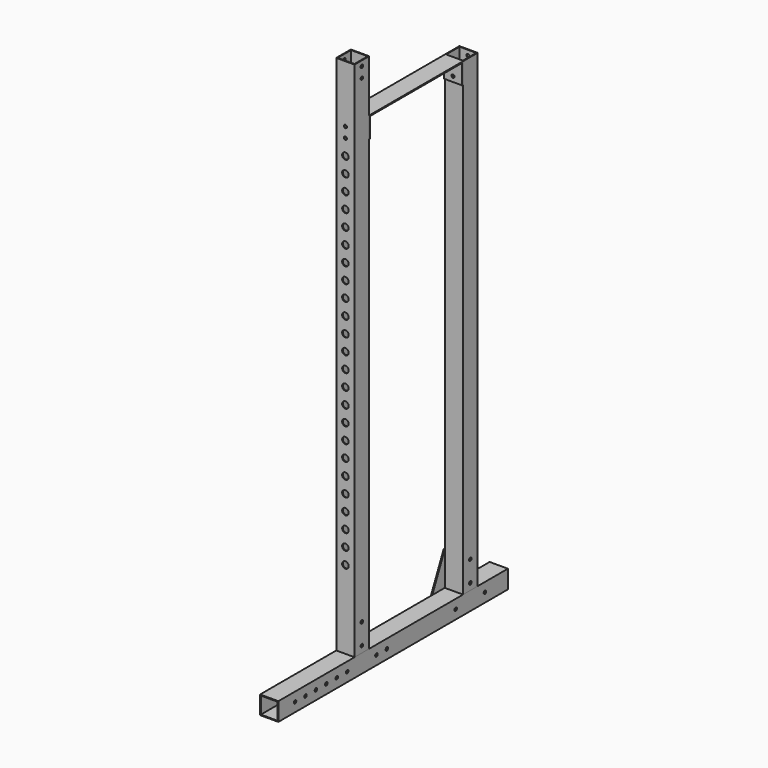
from build123d import *

# Parameters (mm, degrees)
F0_W        = 70
F0_H        = 70
F0_W_2      = 64
F0_H_2      = 64
F1_DEPTH    = 1100
F3_D        = 12
F4_W        = 70
F4_H        = 70
F4_W_2      = 64
F4_H_2      = 64
F5_DEPTH    = 2000
F7_D        = 25
F8_W        = 70
F8_H        = 70
F8_W_2      = 64
F8_H_2      = 64
F9_DEPTH    = 1800
F11_DEPTH   = 70
F13_D       = 12
F13_DEPTH   = 74.001
F13_2_D     = 12
F13_2_DEPTH = 74.001
F15_D       = 12
F15_2_D     = 12
F16_R       = 6
F16_W       = 70
F16_H       = 130
F17_DEPTH   = 4
F19_D       = 12
F21_D       = 12


# Not quite as in the source:
# - a feature names something its author has since deleted; it is built from what else it names


with BuildPart() as f1:
    # F0 (on Front) → F1 (new body)
    with BuildSketch(Plane.XZ):
        with Locations((35, 35)):
            Rectangle(F0_W, F0_H)
        with Locations((35, 35)):
            Rectangle(F0_W_2, F0_H_2, mode=Mode.SUBTRACT)
    extrude(amount=-F1_DEPTH)

    # F3 (through all)
    with Locations(Plane(origin=(0, 0, 0), x_dir=(0, -1, 0), z_dir=(-1, 0, 0))):
        with Locations((-990, 35), (-850, 35), (-520, 35), (-470, 35), (-330, 35), (-280, 35), (-230, 35), (-180, 35), (-130, 35), (-80, 35)):
            Hole(F3_D / 2)


with BuildPart() as f5:
    # F4 (on face) → F5 (new body)
    with BuildSketch(Plane.XY.offset(70)):
        with Locations((35, 400)):
            Rectangle(F4_W, F4_H)
        with Locations((35, 400)):
            Rectangle(F4_W_2, F4_H_2, mode=Mode.SUBTRACT)
    extrude(amount=F5_DEPTH)

    # F7 (through all)
    with Locations(Plane.XZ.offset(-365)):
        with Locations((35, 1510), (35, 1450), (35, 1390), (35, 1330), (35, 1270), (35, 1210), (35, 1150), (35, 1090), (35, 1030), (35, 970), (35, 910), (35, 850), (35, 790), (35, 730), (35, 670), (35, 610), (35, 550), (35, 490), (35, 430), (35, 370), (35, 1570), (35, 1630), (35, 1690), (35, 1750)):
            Hole(F7_D / 2)

    # F15 (through all)
    with Locations(Plane(origin=(0, 439, 0), x_dir=(-1, 0, 0), z_dir=(0, 1, 0))):
        with Locations((-35, 1850), (-35, 1810)):
            Hole(F15_D / 2)

    # F21 (through all)
    with Locations(Plane(origin=(0, 0, 0), x_dir=(0, -1, 0), z_dir=(-1, 0, 0))):
        with Locations((-400, 2050), (-400, 2010), (-400, 175), (-400, 95)):
            Hole(F21_D / 2)


with BuildPart() as f9:
    # F8 (on face) → F9 (new body)
    with BuildSketch(Plane.XY.offset(70)):
        with Locations((35, 920)):
            Rectangle(F8_W, F8_H)
        with Locations((35, 920)):
            Rectangle(F8_W_2, F8_H_2, mode=Mode.SUBTRACT)
    extrude(amount=F9_DEPTH)

    # F13 (through all, one way)
    with BuildSketch(Plane.XZ.offset(-881)):
        with Locations((35, 1850), (35, 1810)):
            Circle(F13_D / 2)
    extrude(amount=-F13_DEPTH, mode=Mode.SUBTRACT)

    # F19 (through all)
    with Locations(Plane(origin=(0, 0, 0), x_dir=(0, -1, 0), z_dir=(-1, 0, 0))):
        with Locations((-920, 175), (-920, 95)):
            Hole(F19_D / 2)


with BuildPart() as f11:
    # F10 (on face) → F11 (new body)
    with BuildSketch(Plane(origin=(0, 0, 0), x_dir=(0, -1, 0), z_dir=(-1, 0, 0))):
        Polygon((-435, 1870), (-885, 1870), (-885, 1790), (-881, 1790), (-881, 1866), (-439, 1866), (-439, 1790), (-435, 1790), align=None)
    extrude(amount=-F11_DEPTH)

    # F13#2 (through all, one way)
    with BuildSketch(Plane.XZ.offset(-881)):
        with Locations((35, 1850), (35, 1810)):
            Circle(F13_2_D / 2)
    extrude(amount=-F13_2_DEPTH, mode=Mode.SUBTRACT)

    # F15#2 (through all)
    with Locations(Plane(origin=(0, 439, 0), x_dir=(-1, 0, 0), z_dir=(0, 1, 0))):
        with Locations((-35, 1850), (-35, 1810)):
            Hole(F15_2_D / 2)


with BuildPart() as f17:
    # F16 (on face) → F17 (new body)
    with BuildSketch(Plane(origin=(0, 0, 0), x_dir=(0, -1, 0), z_dir=(-1, 0, 0))):
        Polygon((-955, 200), (-1015, 70), (-1015, 0), (-825, 0), (-825, 70), (-885, 200), (-885, 70), (-955, 70), align=None)
        with Locations((-990, 35)):
            Circle(F16_R, mode=Mode.SUBTRACT)
        with Locations((-850, 35)):
            Circle(F16_R, mode=Mode.SUBTRACT)
        with Locations((-920, 135)):
            Rectangle(F16_W, F16_H)
        with Locations((-920, 95)):
            Circle(F16_R, mode=Mode.SUBTRACT)
        with Locations((-920, 175)):
            Circle(F16_R, mode=Mode.SUBTRACT)
    extrude(amount=F17_DEPTH)


solid = Compound([f1.part, f5.part, f9.part, f11.part, f17.part])
